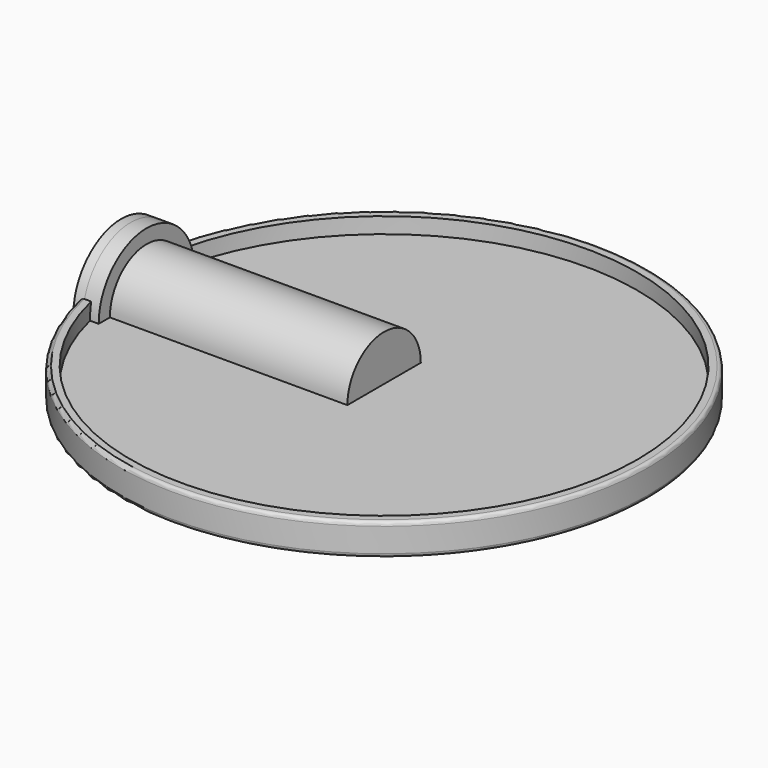
from build123d import *

# Parameters (mm, degrees)
F2_R      = 3.6801131425
F3_DEPTH  = 20.32
F4_R      = 4.8020380174
F4_R_2    = 3.6801131425
F5_DEPTH  = 1.27
F6_R      = 4.8020380174
F6_R_2    = 2.3678967055
F7_DEPTH  = 0.762
F9_R      = 21.1697216963
F9_R_2    = 20.3229858377
F10_DEPTH = 1.27
F8_R      = 21.1697216963
F11_DEPTH = 1.27
F12_R     = 0.3048
F13_DEPTH = 0.762


# Not quite as in the source:
# - the program builds the solid bodies; features that only make, move or delete a surface that nothing else refers to are left out


with BuildPart() as f3:
    # F2 (on Right) → F3 (new body)
    with BuildSketch(Plane.YZ):
        Circle(F2_R)
    extrude(amount=-F3_DEPTH)

    # F4 (on face) → F5 (join)
    with BuildSketch(Plane(origin=(-20.32, 0, 0), x_dir=(0, -1, 0), z_dir=(-1, 0, 0))):
        Circle(F4_R)
        Circle(F4_R_2, mode=Mode.SUBTRACT)
    extrude(amount=-F5_DEPTH)

    # F6 (on face) → F7 (join)
    with BuildSketch(Plane(origin=(-20.32, 0, 0), x_dir=(0, -1, 0), z_dir=(-1, 0, 0))):
        Circle(F6_R)
        Circle(F6_R_2, mode=Mode.SUBTRACT)
    extrude(amount=F7_DEPTH)

    # F9 (on face) → F10 (join)
    with BuildSketch(Plane.XY):
        Circle(F9_R)
        Circle(F9_R_2, mode=Mode.SUBTRACT)
    extrude(amount=F10_DEPTH)

    # F8 (on Top) → F11 (join)
    with BuildSketch(Plane.XY):
        Circle(F8_R)
    extrude(amount=-F11_DEPTH)

    # F12
    f12_edges = [f3.edges().sort_by_distance(p)[0] for p in [
        (21.169722, 0, -1.27),
        (21.169722, 0, 1.27),
    ]]
    fillet(f12_edges, radius=F12_R)

    # F13 (add): faces of the model
    f13_faces = [f3.faces().sort_by_distance(p)[0] for p in [
        (-20.32, 0, -1.7192532993),
        (-20.32, 0, 1.4782041027),
    ]]
    extrude(f13_faces, amount=F13_DEPTH)


solid = f3.part
